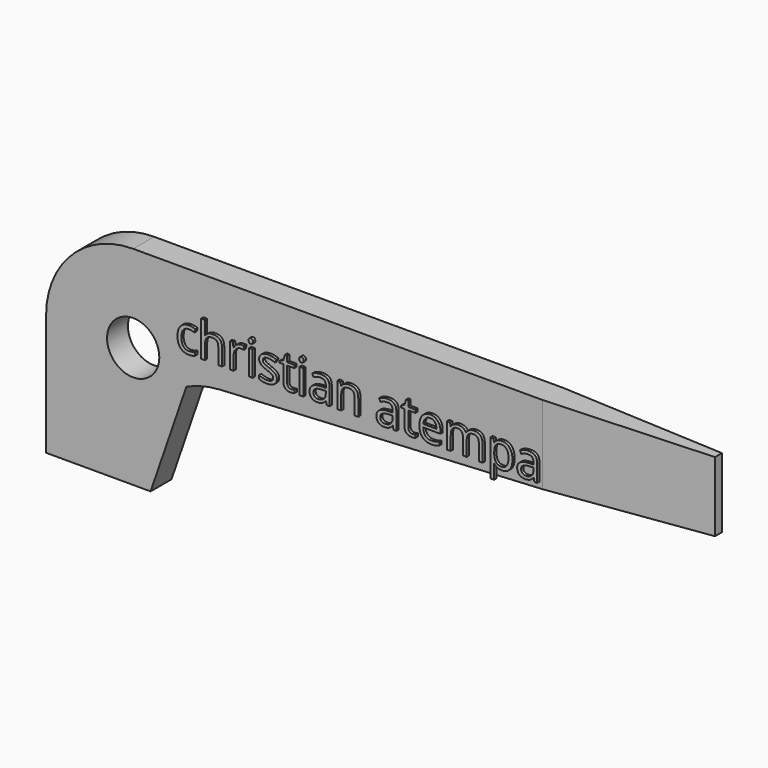
from build123d import *

# Parameters (mm, degrees)
F1_DEPTH     = 2.38125
F2_R         = 2.38125
F3_DEPTH     = 2.38225
F5_DEPTH     = 25.4
F6_TEXT_SIZE = 4.260431284
F7_DEPTH     = 0.254


# Not quite as in the source:
# - Text() gives the source's letters only with a copy of the font that has no kerning and outlines rounded to 1/6400 em; it was checked with that copy


with BuildPart() as f1:
    # F0 (on Front) → F1 (new body)
    with BuildSketch(Plane.XZ):
        with BuildLine():
            Line((60.325, 18.9497377723), (7.9375, 18.9497377723))
            ThreePointArc((7.9375, 18.9497377723), (2.3248399243, 16.624897848), (0, 11.0122377723))
            Line((0, 11.0122377723), (0, 0))
            Line((0, 0), (9.525, 0))
            Line((9.525, 0), (12.7882261162, 9.4748688862))
            ThreePointArc((12.7882261162, 9.4748688862), (14.2969085456, 9.9924802956), (15.875, 10.2241516257))
            Line((15.875, 10.2241516257), (60.325, 12.5997377723))
            Line((60.325, 12.5997377723), (60.325, 18.9497377723))
        make_face()
    extrude(amount=F1_DEPTH)

    # F2 (on face) → F3 (cut, through all)
    with BuildSketch(Plane.XZ.offset(2.38125)):
        with Locations((7.9375, 11.0122377723)):
            Circle(F2_R)
    extrude(amount=-F3_DEPTH, mode=Mode.SUBTRACT)

    # F4 (on face) → F5 (cut)
    with BuildSketch(Plane.XY.offset(18.9497377723)):
        Polygon((60.325, -2.38125), (60.325, -1.5875), (45.24375, -2.38125), align=None)
        Polygon((60.325, 0), (45.24375, 0), (60.325, -0.79375), align=None)
    extrude(amount=-F5_DEPTH, mode=Mode.SUBTRACT)

    # F6 (on face) → F7 (join)
    with BuildSketch(Plane.XZ.offset(2.38125)):
        with Locations((11.9404912069, 12.3042260266)):
            Text('christian atempa', F6_TEXT_SIZE, font='Open Sans', text_align=(TextAlign.LEFT, TextAlign.BOTTOM))
    extrude(amount=F7_DEPTH)


solid = f1.part
